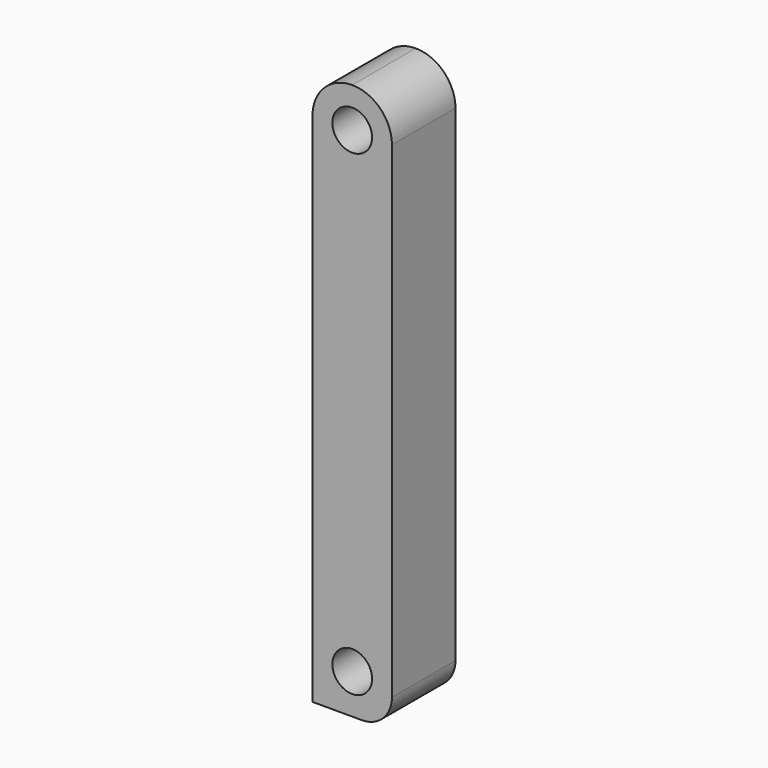
from build123d import *

# Parameters (mm, degrees)
F0_R     = 6.35
F1_DEPTH = 25.4
F2_R     = 12.7
F3_R     = 12.69999


# Not quite as in the source:
# - a fillet or chamfer is up to 0.001 mm smaller than in the source, because OpenCascade refuses the exact size


with BuildPart() as f1:
    # F0 (on Front) → F1 (new body)
    with BuildSketch(Plane.XZ):
        with BuildLine():
            Line((0, 177.8), (0, 0))
            Line((0, 0), (15.8163251287, 0))
            ThreePointArc((15.8163251287, 0), (22.5930066189, 2.8069933811), (25.4, 9.5836748713))
            Line((25.4, 9.5836748713), (25.4, 177.8))
            Line((25.4, 177.8), (0, 177.8))
        make_face()
        with Locations((12.7, 12.7)):
            Circle(F0_R, mode=Mode.SUBTRACT)
        with Locations((12.7, 165.1)):
            Circle(F0_R, mode=Mode.SUBTRACT)
    extrude(amount=F1_DEPTH)

    # F2
    f2_edges = [f1.edges().sort_by_distance(p)[0] for p in [
        (25.4, -12.7, 177.8),
    ]]
    fillet(f2_edges, radius=F2_R)

    # F3 (radius 12.7 in the source; OpenCascade refuses exactly that, so slightly less here)
    f3_edges = [f1.edges().sort_by_distance(p)[0] for p in [
        (0, -12.7, 177.8),
    ]]
    fillet(f3_edges, radius=F3_R)


solid = f1.part
